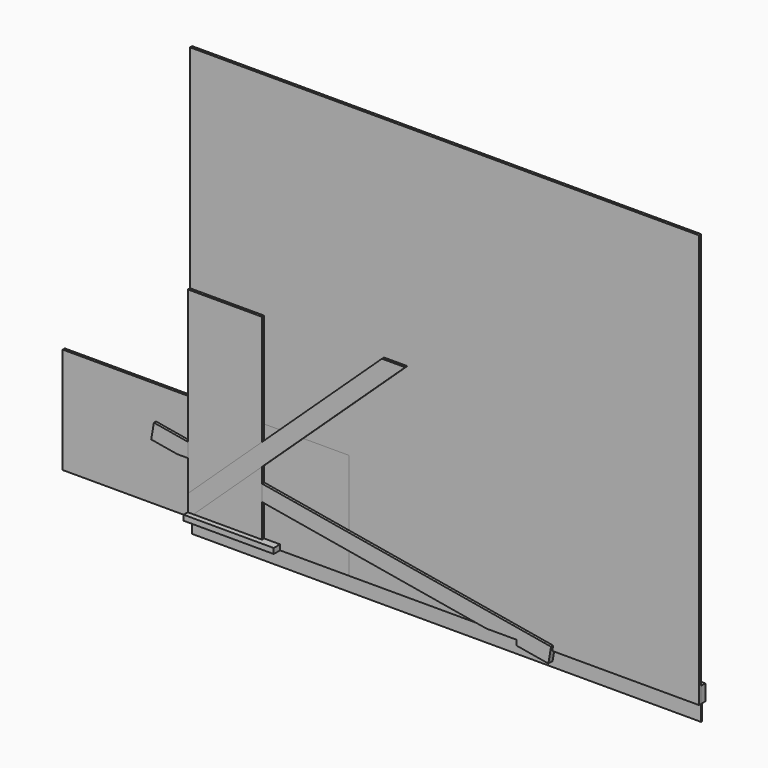
from build123d import *

# Parameters (mm, degrees)
F0_W      = 150
F0_H      = 150
F1_DEPTH  = 3440
F2_W      = 150
F2_H      = 150
F3_DEPTH  = 2940
F4_W      = 50
F4_H      = 150
F5_DEPTH  = 4100
F6_W      = 50
F6_H      = 150
F7_DEPTH  = 3000
F8_W      = 50
F8_H      = 150
F9_DEPTH  = 4800
F10_W     = 150
F10_H     = 20
F11_DEPTH = 4100
F12_W     = 200
F12_H     = 20
F13_DEPTH = 1775
F16_W     = 150
F16_H     = 20
F17_DEPTH = 1975
F19_DEPTH = 50
F21_DEPTH = 4100
F23_DEPTH = 3100
F24_W     = 4800
F24_H     = 3900
F25_DEPTH = 25
F26_W     = 700
F26_H     = 1900
F27_DEPTH = 50
F28_W     = 1500
F28_H     = 1000
F29_DEPTH = 25
F30_W     = 50
F30_H     = 100
F31_DEPTH = 2050
F32_W     = 50
F32_H     = 100
F33_DEPTH = 1900
F34_W     = 50
F34_H     = 100
F35_DEPTH = 800
F36_W     = 50
F36_H     = 100
F37_DEPTH = 700
F38_W     = 100
F38_H     = 50
F39_DEPTH = 1200
F40_W     = 100
F40_H     = 50
F41_DEPTH = 200
F43_DEPTH = 50
F44_W     = 100
F44_H     = 50
F45_DEPTH = 850
F46_W     = 100
F46_H     = 50
F47_DEPTH = 650
F49_DEPTH = 1200
F50_W     = 10
F50_H     = 150
F51_DEPTH = 4800
F52_W     = 1200
F52_H     = 1000
F53_DEPTH = 25


# Not quite as in the source:
# - a feature names something its author has since deleted; it is built from what else it names


with BuildPart() as f1:
    # F0 (on Top) → F1 (new body)
    with BuildSketch(Plane.XY):
        with Locations((75, 75)):
            Rectangle(F0_W, F0_H)
    extrude(amount=F1_DEPTH)


with BuildPart() as f3:
    # F2 (on Top) → F3 (new body)
    with BuildSketch(Plane.XY):
        with Locations((75, 75)):
            Rectangle(F2_W, F2_H)
    extrude(amount=F3_DEPTH)


with BuildPart() as f5:
    # F4 (on Right) → F5 (new body)
    with BuildSketch(Plane.YZ):
        with Locations((25, 75)):
            Rectangle(F4_W, F4_H)
    extrude(amount=F5_DEPTH)


with BuildPart() as f7:
    # F6 (on Right) → F7 (new body)
    with BuildSketch(Plane.YZ):
        with Locations((25, 75)):
            Rectangle(F6_W, F6_H)
    extrude(amount=F7_DEPTH)


with BuildPart() as f9:
    # F8 (on Right) → F9 (new body)
    with BuildSketch(Plane.YZ):
        with Locations((25, 75)):
            Rectangle(F8_W, F8_H)
    extrude(amount=F9_DEPTH)


with BuildPart() as f11:
    # F10 (on Right) → F11 (new body)
    with BuildSketch(Plane.YZ):
        with Locations((75, -10)):
            Rectangle(F10_W, F10_H)
    extrude(amount=F11_DEPTH)


with BuildPart() as f13:
    # F12 (on Right) → F13 (new body)
    with BuildSketch(Plane.YZ):
        with Locations((100, 10)):
            Rectangle(F12_W, F12_H)
    extrude(amount=F13_DEPTH)


with BuildPart() as f14_1:
    # F14: copy of F13
    add(f13.part)


with BuildPart() as f17:
    # F16 (on Right) → F17 (new body)
    with BuildSketch(Plane.YZ):
        with Locations((75, 10)):
            Rectangle(F16_W, F16_H)
    extrude(amount=F17_DEPTH)


with BuildPart() as f19:
    # F18 (on Front) → F19 (new body)
    with BuildSketch(Plane.XZ):
        Polygon((2815.2993068946, 0), (2899.6957839059, 0), (3050, 0), (3100, 0), (3100, -48.8287244524), (3400, -100.2814173698), (3425.3561200039, 47.5599407758), (3396.9886494943, 52.4252166057), (-319.9582863525, 689.9149808739), (-345.3144063564, 542.0736227282), (-100, 500), (0, 500), (50, 500), (50, 474.2736535413), align=None)
    extrude(amount=F19_DEPTH)


with BuildPart() as f21:
    # F20 (on Right) → F21 (new body)
    with BuildSketch(Plane.YZ):
        Polygon((0, 0.6682313415), (10, 0), (20.0011657345, 149.6662175775), (10.0011657345, 150.334448919), align=None)
    extrude(amount=F21_DEPTH)


with BuildPart() as f23:
    # F22 (on Right) → F23 (new body)
    with BuildSketch(Plane.YZ):
        Polygon((0.0222469686, 0.6666666667), (10, 0), (20, 149.666295471), (10.0222469686, 150.3329621376), align=None)
    extrude(amount=F23_DEPTH)


with BuildPart() as f25:
    # F24 (on Front) → F25 (new body)
    with BuildSketch(Plane.XZ):
        with Locations((2400, 1950)):
            Rectangle(F24_W, F24_H)
    extrude(amount=F25_DEPTH)


with BuildPart() as f27:
    # F26 (on Front) → F27 (new body)
    with BuildSketch(Plane.XZ):
        with Locations((350, 950)):
            Rectangle(F26_W, F26_H)
    extrude(amount=F27_DEPTH)


with BuildPart() as f29:
    # F28 (on Front) → F29 (new body)
    with BuildSketch(Plane.XZ):
        with Locations((750, 500)):
            Rectangle(F28_W, F28_H)
    extrude(amount=F29_DEPTH)


with BuildPart() as f31:
    # F30 (on Top) → F31 (new body)
    with BuildSketch(Plane.XY):
        with Locations((25, 50)):
            Rectangle(F30_W, F30_H)
    extrude(amount=F31_DEPTH)


with BuildPart() as f33:
    # F32 (on Top) → F33 (new body)
    with BuildSketch(Plane.XY):
        with Locations((25, 50)):
            Rectangle(F32_W, F32_H)
    extrude(amount=F33_DEPTH)


with BuildPart() as f35:
    # F34 (on Right) → F35 (new body)
    with BuildSketch(Plane.YZ):
        with Locations((25, 50)):
            Rectangle(F34_W, F34_H)
    extrude(amount=F35_DEPTH)


with BuildPart() as f37:
    # F36 (on Top) → F37 (new body)
    with BuildSketch(Plane.XY):
        with Locations((-25, 50)):
            Rectangle(F36_W, F36_H)
    extrude(amount=F37_DEPTH)


with BuildPart() as f39:
    # F38 (on Right) → F39 (new body)
    with BuildSketch(Plane.YZ):
        with Locations((50, 25)):
            Rectangle(F38_W, F38_H)
    extrude(amount=F39_DEPTH)


with BuildPart() as f41:
    # F40 (on Right) → F41 (new body)
    with BuildSketch(Plane.YZ):
        with Locations((50, 25)):
            Rectangle(F40_W, F40_H)
    extrude(amount=F41_DEPTH)


with BuildPart() as f43:
    # F42 (on Front) → F43 (new body)
    with BuildSketch(Plane.XZ):
        Polygon((2050, 1920), (1830.5688617947, 1920), (0, 205.5159928557), (0, 0), align=None)
    extrude(amount=F43_DEPTH)


with BuildPart() as f45:
    # F44 (on Right) → F45 (new body)
    with BuildSketch(Plane.YZ):
        with Locations((-50, 25)):
            Rectangle(F44_W, F44_H)
    extrude(amount=F45_DEPTH)


with BuildPart() as f47:
    # F46 (on Right) → F47 (new body)
    with BuildSketch(Plane.YZ):
        with Locations((50, 25)):
            Rectangle(F46_W, F46_H)
    extrude(amount=F47_DEPTH)


with BuildPart() as f49:
    # F48 (on Right) → F49 (new body)
    with BuildSketch(Plane.YZ):
        Polygon((0, 0.6681531048), (10, 0), (20, 149.666295471), (10, 150.3344485757), align=None)
    extrude(amount=F49_DEPTH)


with BuildPart() as f51:
    # F50 (on Right) → F51 (new body)
    with BuildSketch(Plane.YZ):
        with Locations((5, -75)):
            Rectangle(F50_W, F50_H)
    extrude(amount=F51_DEPTH)


with BuildPart() as f53:
    # F52 (on Front) → F53 (new body)
    with BuildSketch(Plane.XZ):
        with Locations((-600, 500)):
            Rectangle(F52_W, F52_H)
    extrude(amount=F53_DEPTH)


solid = Compound([f1.part, f3.part, f5.part, f7.part, f9.part, f11.part, f13.part, f17.part, f19.part, f21.part, f23.part, f25.part, f27.part, f29.part, f31.part, f33.part, f35.part, f37.part, f39.part, f41.part, f43.part, f45.part, f47.part, f49.part, f51.part, f53.part])
